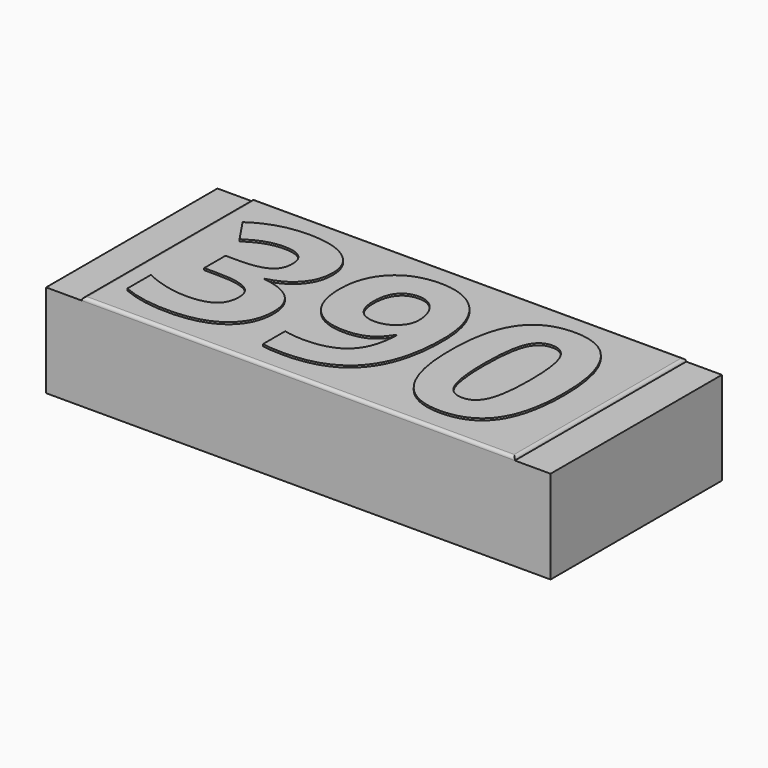
from build123d import *

# Parameters (mm, degrees)
F0_W         = 3.25
F0_H         = 1.38
F1_DEPTH     = 0.6
F2_W         = 2.79
F2_H         = 1.38
F3_DEPTH     = 0.02
F4_R         = 0.01999
F5_TEXT_SIZE = 1.4821604054
F6_DEPTH     = 0.0125


# Not quite as in the source:
# - a fillet or chamfer is up to 0.001 mm smaller than in the source, because OpenCascade refuses the exact size
# - Text() gives the source's letters only with a copy of the font that has no kerning and outlines rounded to 1/6400 em; it was checked with that copy


with BuildPart() as f1:
    # F0 (on Top) → F1 (new body)
    with BuildSketch(Plane.XY):
        with Locations((1.625, 0.69)):
            Rectangle(F0_W, F0_H)
    extrude(amount=F1_DEPTH)


with BuildPart() as f3:
    # F2 (on face) → F3 (new body)
    with BuildSketch(Plane.XY.offset(0.6)):
        with Locations((1.6248731415, 0.69)):
            Rectangle(F2_W, F2_H)
    extrude(amount=F3_DEPTH)

    # F4 (radius 0.02 in the source; OpenCascade refuses exactly that, so slightly less here)
    f4_edges = [f3.edges().sort_by_distance(p)[0] for p in [
        (1.624873, 1.38, 0.62),
        (0.229873, 0.69, 0.62),
        (1.624873, 0, 0.62),
        (3.019873, 0.69, 0.62),
    ]]
    fillet(f4_edges, radius=F4_R)


with BuildPart() as f6:
    # F5 (on face) → F6 (new body)
    with BuildSketch(Plane.XY.offset(0.62)):
        with Locations((0.3090505779, 0.154741123)):
            Text('390', F5_TEXT_SIZE, font='Open Sans', font_style=FontStyle.BOLD, text_align=(TextAlign.LEFT, TextAlign.BOTTOM))
    extrude(amount=F6_DEPTH)


solid = Compound([f1.part, f3.part, f6.part])
